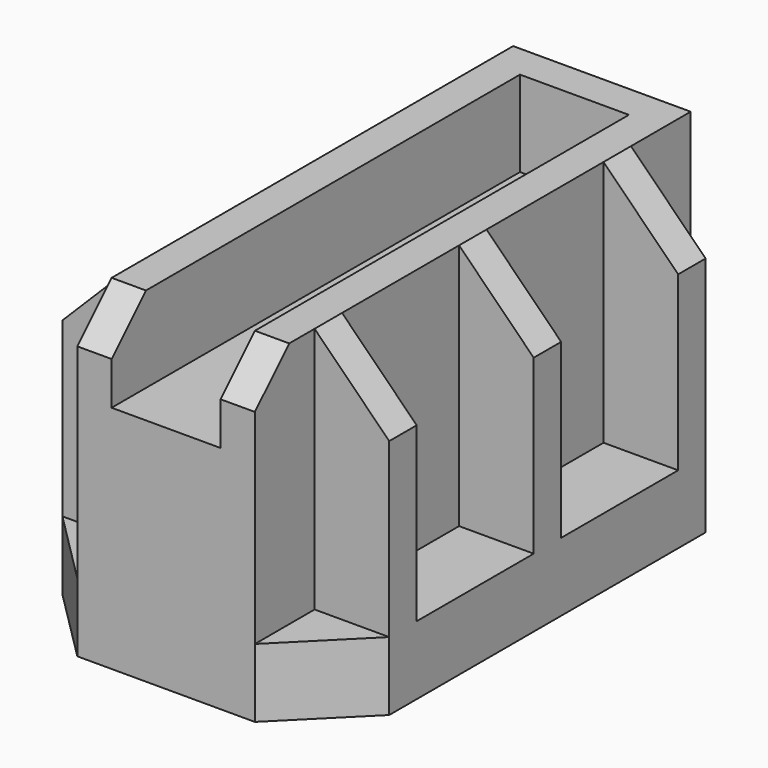
from build123d import *

# Parameters (mm, degrees)
F1_DEPTH  = 31.75
F2_T      = -4
F3_W      = 4
F3_H      = 10
F4_DEPTH  = 63.5
F6_DEPTH  = 8
F8_DEPTH  = 2
F11_DEPTH = 4
F13_DEPTH = 4
F14_W     = 12.7
F14_H     = 4
F15_DEPTH = 10
F16_SIZE  = 5
F17_R     = 2.15
F18_DEPTH = 25
F19_W     = 30.1
F19_H     = 4


# Not quite as in the source:
# - a pattern or mirror of a feature is missing from the dataset's text; its kind, count and spacing are read off the source's solid


with BuildPart() as f1:
    # F0 (on Front) → F1 (new body, symmetric)
    with BuildSketch(Plane.XZ):
        Polygon((-10.35, 0), (10.35, 0), (10.35, 26.81), (6.35, 26.81), (-6.35, 26.81), (-10.35, 26.81), align=None)
    extrude(amount=F1_DEPTH, both=True)

    # F2
    f2_openings = [f1.faces().sort_by_distance(p)[0] for p in [
        (0, 0, 0),
    ]]
    offset(amount=F2_T, openings=f2_openings)

    # F3 (on face) → F4 (join, through all)
    with BuildSketch(Plane.XZ.offset(31.75)):
        with Locations((-8.35, 31.81)):
            Rectangle(F3_W, F3_H)
        with Locations((8.35, 31.81)):
            Rectangle(F3_W, F3_H)
    extrude(amount=-F4_DEPTH)

    # F5 (on Top) → F6 (join)
    with BuildSketch(Plane.XY):
        Polygon((-19.05, -23.05), (-10.35, -31.75), (-10.35, 31.75), (-19.05, 23.05), align=None)
        Polygon((10.35, 31.75), (10.35, -31.75), (19.05, -23.05), (19.05, 23.05), align=None)
    extrude(amount=F6_DEPTH)

    # F7 (on Front) → F8 (join, symmetric)
    with BuildSketch(Plane.XZ):
        Polygon((-19.05, 8), (-10.35, 8), (-10.35, 36.81), (-19.05, 28.11), align=None)
        Polygon((10.35, 8), (19.05, 8), (19.05, 28.11), (10.35, 36.81), align=None)
    f8 = extrude(amount=F8_DEPTH, both=True)

    # F8_copies: F8 across plane
    add(f8.mirror(Plane(origin=(0, -10.525, 0), x_dir=(0, 0, -1), z_dir=(0, -1, 0))))

    # F10 (on plane+point) → F11 (join)
    with BuildSketch(Plane.XZ.offset(-23.05)):
        Polygon((10.35, 8), (19.05, 8), (19.05, 28.11), (10.35, 36.81), align=None)
        Polygon((-19.05, 28.11), (-19.05, 8), (-10.35, 8), (-10.35, 36.81), align=None)
    extrude(amount=F11_DEPTH)

    # F12 (on face) → F13 (cut)
    with BuildSketch(Plane(origin=(0, 0, 0), x_dir=(1, 0, 0), z_dir=(0, 0, -1))):
        Polygon((-8.6931457505, -27.75), (8.6931457505, -27.75), (15.05, -21.3931457505), (15.05, 21.3931457505), (8.6931457505, 27.75), (-8.6931457505, 27.75), (-15.05, 21.3931457505), (-15.05, -21.3931457505), align=None)
    extrude(amount=-F13_DEPTH, mode=Mode.SUBTRACT)

    # F14 (on face) → F15 (join, through all)
    with BuildSketch(Plane.XY.offset(26.81)):
        with Locations((0, 29.75)):
            Rectangle(F14_W, F14_H)
    extrude(amount=F15_DEPTH)

    # F16
    f16_edges = [f1.edges().sort_by_distance(p)[0] for p in [
        (8.35, -31.75, 36.81),
        (-8.35, -31.75, 36.81),
    ]]
    chamfer(f16_edges, length=F16_SIZE)

    # F17 (on face) → F18 (cut)
    with BuildSketch(Plane.XY.offset(26.81)):
        with Locations((0, -10.525)):
            Circle(F17_R)
    extrude(amount=-F18_DEPTH, mode=Mode.SUBTRACT)

    # F19 (on face) → F20 (join, up to the next surface of F1)
    with BuildSketch(Plane(origin=(0, 0, 0), x_dir=(1, 0, 0), z_dir=(0, 0, -1))):
        with Locations((0, -10.525)):
            Rectangle(F19_W, F19_H)
    extrude(until=Until.NEXT, dir=(0, 0, 1))


solid = f1.part
